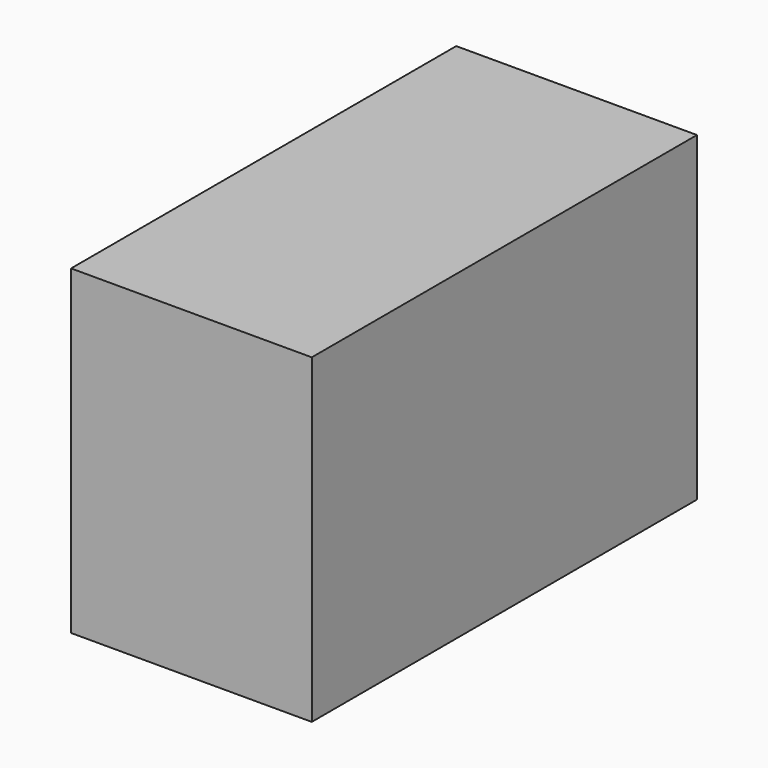
from build123d import *

# Parameters (mm, degrees)
F0_W     = 76.2
F0_H     = 101.6
F1_DEPTH = 76.2


# Not quite as in the source:
# - the program builds the solid bodies; features that only make, move or delete a surface that nothing else refers to are left out


with BuildPart() as f1:
    # F0 (on Front) → F1 (new body, symmetric)
    with BuildSketch(Plane.XZ):
        with Locations((69.984262497, 96.8042679829)):
            Rectangle(F0_W, F0_H)
    extrude(amount=F1_DEPTH, both=True)


solid = f1.part
